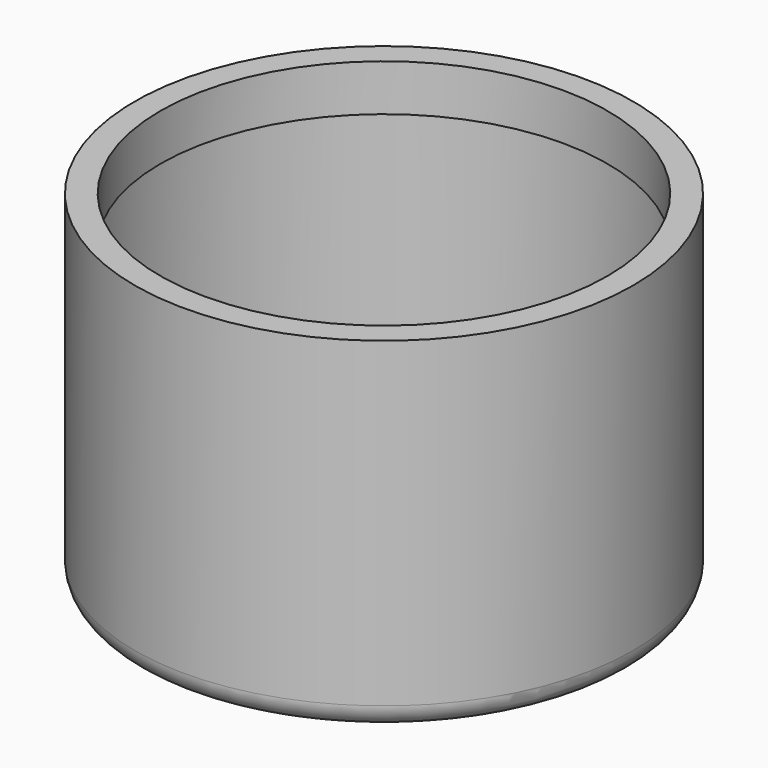
from build123d import *

# Parameters (mm, degrees)
F0_R          = 52.5
F0_R_2        = 50.5
F0_R_3        = 47.5
F1_DEPTH      = 10
F1_DEPTH_BACK = 4
F0_R_4        = 53.5
F2_DEPTH      = 70
F2_DEPTH_BACK = 4
F4_R          = 52.5
F4_R_2        = 48
F5_DEPTH      = 10
F8_R          = 5


# Not quite as in the source:
# - the program builds the solid bodies; features that only make, move or delete a surface that nothing else refers to are left out


with BuildPart() as f1:
    # F0 (on Top) → F1 (new body, two sides)
    with BuildSketch(Plane.XY) as f1_sk:
        Circle(F0_R)
        Circle(F0_R_2, mode=Mode.SUBTRACT)
        Circle(F0_R_2)
        Circle(F0_R_3, mode=Mode.SUBTRACT)
    extrude(amount=F1_DEPTH)
    extrude(f1_sk.sketch, amount=-F1_DEPTH_BACK)

    # F0 (on Top) → F2 (join, two sides)
    with BuildSketch(Plane.XY) as f2_sk:
        Circle(F0_R_4)
        Circle(F0_R, mode=Mode.SUBTRACT)
    extrude(amount=F2_DEPTH)
    extrude(f2_sk.sketch, amount=-F2_DEPTH_BACK)

    # F4 (on offset) → F5 (join)
    with BuildSketch(Plane.XY.offset(60)):
        Circle(F4_R)
        Circle(F4_R_2, mode=Mode.SUBTRACT)
    extrude(amount=F5_DEPTH)

    # F8
    f8_edges = [f1.edges().sort_by_distance(p)[0] for p in [
        (-53.5, 0, -4),
    ]]
    fillet(f8_edges, radius=F8_R)


solid = f1.part
